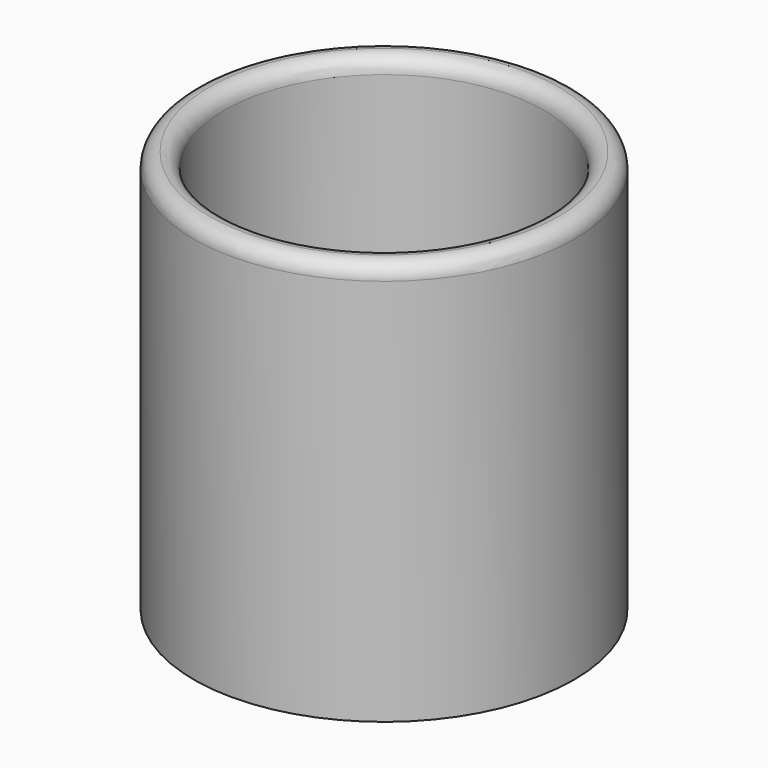
from build123d import *

# Parameters (mm, degrees)
F0_R     = 25
F1_DEPTH = 3
F2_R     = 25
F2_R_2   = 21
F3_DEPTH = 50
F4_R     = 1.99999


# Not quite as in the source:
# - a fillet or chamfer is up to 0.001 mm smaller than in the source, because OpenCascade refuses the exact size


with BuildPart() as f1:
    # F0 (on Top) → F1 (new body)
    with BuildSketch(Plane.XY):
        Circle(F0_R)
    extrude(amount=F1_DEPTH)

    # F2 (on face) → F3 (join)
    with BuildSketch(Plane.XY.offset(3)):
        Circle(F2_R)
        Circle(F2_R_2, mode=Mode.SUBTRACT)
    extrude(amount=F3_DEPTH)

    # F4 (radius 2 in the source; OpenCascade refuses exactly that, so slightly less here)
    f4_edges = [f1.edges().sort_by_distance(p)[0] for p in [
        (-25, 0, 53),
        (-21, 0, 53),
    ]]
    fillet(f4_edges, radius=F4_R)


solid = f1.part
